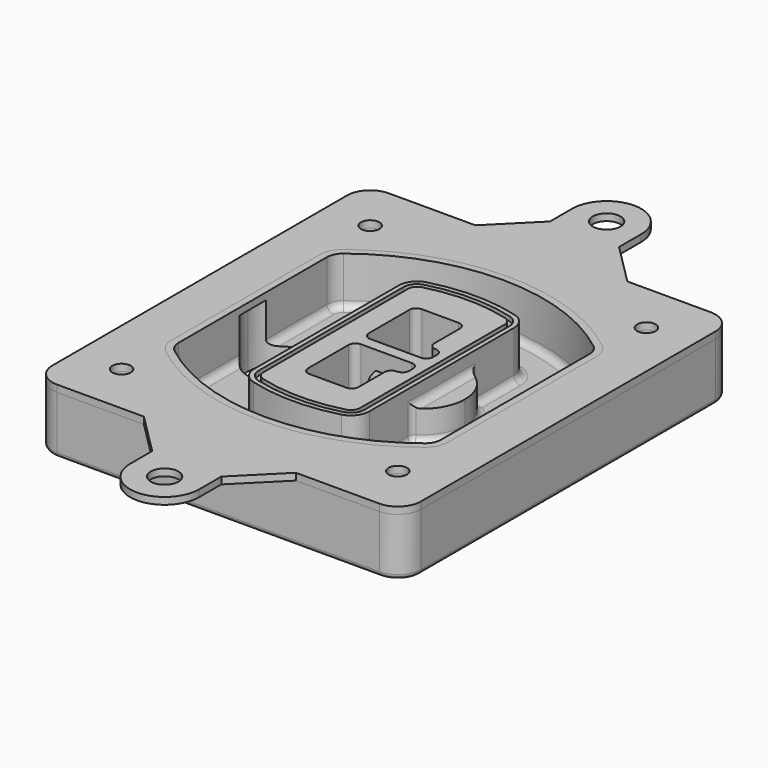
from build123d import *

# Parameters (mm, degrees)
F0_R      = 4
F1_DEPTH  = 25
F2_DEPTH  = 3
F3_DEPTH  = 18
F5_DEPTH  = 21
F6_DEPTH  = 2
F8_DEPTH  = 20
F9_DEPTH  = 16
F10_DEPTH = 25
F7_R      = 6
F7_R_2    = 4
F11_DEPTH = 6
F13_DEPTH = 9
F14_R     = 3
F15_R     = 2
F16_R     = 6
F16_R_2   = 4
F17_DEPTH = 3


with BuildPart() as f1:
    # F0 (on Top) → F1 (new body)
    with BuildSketch(Plane.XY):
        with BuildLine():
            ThreePointArc((14.05, 38.3825811321), (16.9789321881, 31.3115133202), (24.05, 28.3825811321))
            Line((24.05, 28.3825811321), (164.05, 28.3825811321))
            ThreePointArc((164.05, 28.3825811321), (171.1210678119, 31.3115133202), (174.05, 38.3825811321))
            Line((174.05, 38.3825811321), (174.05, 198.3825811321))
            ThreePointArc((174.05, 198.3825811321), (171.1210678119, 205.4536489439), (164.05, 208.3825811321))
            Line((164.05, 208.3825811321), (24.05, 208.3825811321))
            ThreePointArc((24.05, 208.3825811321), (16.9789321881, 205.4536489439), (14.05, 198.3825811321))
            Line((14.05, 198.3825811321), (14.05, 38.3825811321))
        make_face()
        with Locations((34.05, 50.8825811321)):
            Circle(F0_R, mode=Mode.SUBTRACT)
        with Locations((154.05, 50.8825811321)):
            Circle(F0_R, mode=Mode.SUBTRACT)
        with BuildLine():
            ThreePointArc((30.05, 158.6760234193), (31.4679615202, 164.8154295545), (35.4346153846, 169.7112011673))
            ThreePointArc((35.4346153846, 169.7112011673), (94.05, 189.8825811321), (152.6653846154, 169.7112011673))
            ThreePointArc((152.6653846154, 169.7112011673), (156.6320384798, 164.8154295545), (158.05, 158.6760234193))
            Line((158.05, 158.6760234193), (158.05, 78.0891388448))
            ThreePointArc((158.05, 78.0891388448), (156.6320384798, 71.9497327097), (152.6653846154, 67.0539610969))
            ThreePointArc((152.6653846154, 67.0539610969), (94.05, 46.8825811321), (35.4346153846, 67.0539610969))
            ThreePointArc((35.4346153846, 67.0539610969), (31.4679615202, 71.9497327097), (30.05, 78.0891388448))
            Line((30.05, 78.0891388448), (30.05, 158.6760234193))
        make_face(mode=Mode.SUBTRACT)
        with Locations((34.05, 185.8825811321)):
            Circle(F0_R, mode=Mode.SUBTRACT)
        with Locations((154.05, 185.8825811321)):
            Circle(F0_R, mode=Mode.SUBTRACT)
        with BuildLine():
            ThreePointArc((152.6653846154, 169.7112011673), (94.05, 189.8825811321), (35.4346153846, 169.7112011673))
            ThreePointArc((35.4346153846, 169.7112011673), (31.4679615202, 164.8154295545), (30.05, 158.6760234193))
            Line((30.05, 158.6760234193), (30.05, 78.0891388448))
            ThreePointArc((30.05, 78.0891388448), (31.4679615202, 71.9497327097), (35.4346153846, 67.0539610969))
            ThreePointArc((35.4346153846, 67.0539610969), (94.05, 46.8825811321), (152.6653846154, 67.0539610969))
            ThreePointArc((152.6653846154, 67.0539610969), (156.6320384798, 71.9497327097), (158.05, 78.0891388448))
            Line((158.05, 78.0891388448), (158.05, 158.6760234193))
            ThreePointArc((158.05, 158.6760234193), (156.6320384798, 164.8154295545), (152.6653846154, 169.7112011673))
        make_face()
        with BuildLine():
            Line((34.05, 78.0891388448), (34.05, 158.6760234193))
            ThreePointArc((34.05, 158.6760234193), (35.0628296573, 163.0613135158), (37.8961538462, 166.5582932393))
            ThreePointArc((37.8961538462, 166.5582932393), (94.05, 185.8825811321), (150.2038461538, 166.5582932393))
            ThreePointArc((150.2038461538, 166.5582932393), (153.0371703427, 163.0613135158), (154.05, 158.6760234193))
            Line((154.05, 158.6760234193), (154.05, 78.0891388448))
            ThreePointArc((154.05, 78.0891388448), (153.0371703427, 73.7038487483), (150.2038461538, 70.2068690248))
            ThreePointArc((150.2038461538, 70.2068690248), (94.05, 50.8825811321), (37.8961538462, 70.2068690248))
            ThreePointArc((37.8961538462, 70.2068690248), (35.0628296573, 73.7038487483), (34.05, 78.0891388448))
        make_face(mode=Mode.SUBTRACT)
        with BuildLine():
            ThreePointArc((37.8961538462, 166.5582932393), (35.0628296573, 163.0613135158), (34.05, 158.6760234193))
            Line((34.05, 158.6760234193), (34.05, 78.0891388448))
            ThreePointArc((34.05, 78.0891388448), (35.0628296573, 73.7038487483), (37.8961538462, 70.2068690248))
            ThreePointArc((37.8961538462, 70.2068690248), (94.05, 50.8825811321), (150.2038461538, 70.2068690248))
            ThreePointArc((150.2038461538, 70.2068690248), (153.0371703427, 73.7038487483), (154.05, 78.0891388448))
            Line((154.05, 78.0891388448), (154.05, 158.6760234193))
            ThreePointArc((154.05, 158.6760234193), (153.0371703427, 163.0613135158), (150.2038461538, 166.5582932393))
            ThreePointArc((150.2038461538, 166.5582932393), (94.05, 185.8825811321), (37.8961538462, 166.5582932393))
        make_face()
        with BuildLine():
            ThreePointArc((148.3576923077, 164.1936122933), (150.3410192399, 161.7457264869), (151.05, 158.6760234193))
            Line((151.05, 158.6760234193), (151.05, 78.0891388448))
            ThreePointArc((151.05, 78.0891388448), (150.3410192399, 75.0194357772), (148.3576923077, 72.5715499708))
            ThreePointArc((148.3576923077, 72.5715499708), (94.05, 53.8825811321), (39.7423076923, 72.5715499708))
            ThreePointArc((39.7423076923, 72.5715499708), (37.7589807601, 75.0194357772), (37.05, 78.0891388448))
            Line((37.05, 78.0891388448), (37.05, 158.6760234193))
            ThreePointArc((37.05, 158.6760234193), (37.7589807601, 161.7457264869), (39.7423076923, 164.1936122933))
            ThreePointArc((39.7423076923, 164.1936122933), (94.05, 182.8825811321), (148.3576923077, 164.1936122933))
        make_face(mode=Mode.SUBTRACT)
        with BuildLine():
            Line((151.05, 78.0891388448), (151.05, 158.6760234193))
            ThreePointArc((151.05, 158.6760234193), (150.3410192399, 161.7457264869), (148.3576923077, 164.1936122933))
            ThreePointArc((148.3576923077, 164.1936122933), (94.05, 182.8825811321), (39.7423076923, 164.1936122933))
            ThreePointArc((39.7423076923, 164.1936122933), (37.7589807601, 161.7457264869), (37.05, 158.6760234193))
            Line((37.05, 158.6760234193), (37.05, 78.0891388448))
            ThreePointArc((37.05, 78.0891388448), (37.7589807601, 75.0194357772), (39.7423076923, 72.5715499708))
            ThreePointArc((39.7423076923, 72.5715499708), (94.05, 53.8825811321), (148.3576923077, 72.5715499708))
            ThreePointArc((148.3576923077, 72.5715499708), (150.3410192399, 75.0194357772), (151.05, 78.0891388448))
        make_face()
    extrude(amount=-F1_DEPTH)

    # F0 (on Top) → F2 (join)
    with BuildSketch(Plane.XY):
        with BuildLine():
            ThreePointArc((37.8961538462, 166.5582932393), (35.0628296573, 163.0613135158), (34.05, 158.6760234193))
            Line((34.05, 158.6760234193), (34.05, 78.0891388448))
            ThreePointArc((34.05, 78.0891388448), (35.0628296573, 73.7038487483), (37.8961538462, 70.2068690248))
            ThreePointArc((37.8961538462, 70.2068690248), (94.05, 50.8825811321), (150.2038461538, 70.2068690248))
            ThreePointArc((150.2038461538, 70.2068690248), (153.0371703427, 73.7038487483), (154.05, 78.0891388448))
            Line((154.05, 78.0891388448), (154.05, 158.6760234193))
            ThreePointArc((154.05, 158.6760234193), (153.0371703427, 163.0613135158), (150.2038461538, 166.5582932393))
            ThreePointArc((150.2038461538, 166.5582932393), (94.05, 185.8825811321), (37.8961538462, 166.5582932393))
        make_face()
        with BuildLine():
            ThreePointArc((148.3576923077, 164.1936122933), (150.3410192399, 161.7457264869), (151.05, 158.6760234193))
            Line((151.05, 158.6760234193), (151.05, 78.0891388448))
            ThreePointArc((151.05, 78.0891388448), (150.3410192399, 75.0194357772), (148.3576923077, 72.5715499708))
            ThreePointArc((148.3576923077, 72.5715499708), (94.05, 53.8825811321), (39.7423076923, 72.5715499708))
            ThreePointArc((39.7423076923, 72.5715499708), (37.7589807601, 75.0194357772), (37.05, 78.0891388448))
            Line((37.05, 78.0891388448), (37.05, 158.6760234193))
            ThreePointArc((37.05, 158.6760234193), (37.7589807601, 161.7457264869), (39.7423076923, 164.1936122933))
            ThreePointArc((39.7423076923, 164.1936122933), (94.05, 182.8825811321), (148.3576923077, 164.1936122933))
        make_face(mode=Mode.SUBTRACT)
    extrude(amount=F2_DEPTH)

    # F0 (on Top) → F3 (cut)
    with BuildSketch(Plane.XY):
        with BuildLine():
            Line((151.05, 78.0891388448), (151.05, 158.6760234193))
            ThreePointArc((151.05, 158.6760234193), (150.3410192399, 161.7457264869), (148.3576923077, 164.1936122933))
            ThreePointArc((148.3576923077, 164.1936122933), (94.05, 182.8825811321), (39.7423076923, 164.1936122933))
            ThreePointArc((39.7423076923, 164.1936122933), (37.7589807601, 161.7457264869), (37.05, 158.6760234193))
            Line((37.05, 158.6760234193), (37.05, 78.0891388448))
            ThreePointArc((37.05, 78.0891388448), (37.7589807601, 75.0194357772), (39.7423076923, 72.5715499708))
            ThreePointArc((39.7423076923, 72.5715499708), (94.05, 53.8825811321), (148.3576923077, 72.5715499708))
            ThreePointArc((148.3576923077, 72.5715499708), (150.3410192399, 75.0194357772), (151.05, 78.0891388448))
        make_face()
    extrude(amount=-F3_DEPTH, mode=Mode.SUBTRACT)

    # F4 (on face) → F5 (join, through all)
    with BuildSketch(Plane.XY.offset(3)):
        with BuildLine():
            ThreePointArc((69.05, 79.13605345), (70.6988454002, 74.2716074127), (74.9657088123, 71.4123412437))
            ThreePointArc((74.9657088123, 71.4123412437), (94.05, 68.8825811321), (113.1342911877, 71.4123412437))
            ThreePointArc((113.1342911877, 71.4123412437), (117.4011545998, 74.2716074127), (119.05, 79.13605345))
            Line((119.05, 79.13605345), (119.05, 157.6291088141))
            ThreePointArc((119.05, 157.6291088141), (117.4011545998, 162.4935548514), (113.1342911877, 165.3528210204))
            ThreePointArc((113.1342911877, 165.3528210204), (94.05, 167.8825811321), (74.9657088123, 165.3528210204))
            ThreePointArc((74.9657088123, 165.3528210204), (70.6988454002, 162.4935548514), (69.05, 157.6291088141))
            Line((69.05, 157.6291088141), (69.05, 79.13605345))
        make_face()
        with BuildLine():
            ThreePointArc((112.6132183908, 163.4218929688), (115.8133659499, 161.2774433421), (117.05, 157.6291088141))
            Line((117.05, 157.6291088141), (117.05, 79.13605345))
            ThreePointArc((117.05, 79.13605345), (115.8133659499, 75.4877189221), (112.6132183908, 73.3432692953))
            ThreePointArc((112.6132183908, 73.3432692953), (94.05, 70.8825811321), (75.4867816092, 73.3432692953))
            ThreePointArc((75.4867816092, 73.3432692953), (72.2866340501, 75.4877189221), (71.05, 79.13605345))
            Line((71.05, 79.13605345), (71.05, 157.6291088141))
            ThreePointArc((71.05, 157.6291088141), (72.2866340501, 161.2774433421), (75.4867816092, 163.4218929688))
            ThreePointArc((75.4867816092, 163.4218929688), (94.05, 165.8825811321), (112.6132183908, 163.4218929688))
        make_face(mode=Mode.SUBTRACT)
        with BuildLine():
            Line((117.05, 79.13605345), (117.05, 157.6291088141))
            ThreePointArc((117.05, 157.6291088141), (115.8133659499, 161.2774433421), (112.6132183908, 163.4218929688))
            ThreePointArc((112.6132183908, 163.4218929688), (94.05, 165.8825811321), (75.4867816092, 163.4218929688))
            ThreePointArc((75.4867816092, 163.4218929688), (72.2866340501, 161.2774433421), (71.05, 157.6291088141))
            Line((71.05, 157.6291088141), (71.05, 79.13605345))
            ThreePointArc((71.05, 79.13605345), (72.2866340501, 75.4877189221), (75.4867816092, 73.3432692953))
            ThreePointArc((75.4867816092, 73.3432692953), (94.05, 70.8825811321), (112.6132183908, 73.3432692953))
            ThreePointArc((112.6132183908, 73.3432692953), (115.8133659499, 75.4877189221), (117.05, 79.13605345))
        make_face()
        with BuildLine():
            ThreePointArc((112.0921455939, 161.4909649173), (114.2255772999, 160.0613318328), (115.05, 157.6291088141))
            Line((115.05, 157.6291088141), (115.05, 79.13605345))
            ThreePointArc((115.05, 79.13605345), (114.2255772999, 76.7038304314), (112.0921455939, 75.2741973469))
            ThreePointArc((112.0921455939, 75.2741973469), (94.05, 72.8825811321), (76.0078544061, 75.2741973469))
            ThreePointArc((76.0078544061, 75.2741973469), (73.8744227001, 76.7038304314), (73.05, 79.13605345))
            Line((73.05, 79.13605345), (73.05, 157.6291088141))
            ThreePointArc((73.05, 157.6291088141), (73.8744227001, 160.0613318328), (76.0078544061, 161.4909649173))
            ThreePointArc((76.0078544061, 161.4909649173), (94.05, 163.8825811321), (112.0921455939, 161.4909649173))
        make_face(mode=Mode.SUBTRACT)
        with BuildLine():
            Line((115.05, 79.13605345), (115.05, 157.6291088141))
            ThreePointArc((115.05, 157.6291088141), (114.2255772999, 160.0613318328), (112.0921455939, 161.4909649173))
            ThreePointArc((112.0921455939, 161.4909649173), (94.05, 163.8825811321), (76.0078544061, 161.4909649173))
            ThreePointArc((76.0078544061, 161.4909649173), (73.8744227001, 160.0613318328), (73.05, 157.6291088141))
            Line((73.05, 157.6291088141), (73.05, 79.13605345))
            ThreePointArc((73.05, 79.13605345), (73.8744227001, 76.7038304314), (76.0078544061, 75.2741973469))
            ThreePointArc((76.0078544061, 75.2741973469), (94.05, 72.8825811321), (112.0921455939, 75.2741973469))
            ThreePointArc((112.0921455939, 75.2741973469), (114.2255772999, 76.7038304314), (115.05, 79.13605345))
        make_face()
        with BuildLine():
            Line((86.05, 115.8825811321), (108.05, 115.8825811321))
            ThreePointArc((108.05, 115.8825811321), (110.1713203436, 115.0039014756), (111.05, 112.8825811321))
            Line((111.05, 112.8825811321), (111.05, 110.8825811321))
            ThreePointArc((111.05, 110.8825811321), (110.1713203436, 108.7612607885), (108.05, 107.8825811321))
            ThreePointArc((108.05, 107.8825811321), (105.9286796564, 107.0039014756), (105.05, 104.8825811321))
            Line((105.05, 104.8825811321), (105.05, 90.8825811321))
            ThreePointArc((105.05, 90.8825811321), (104.1713203436, 88.7612607885), (102.05, 87.8825811321))
            Line((102.05, 87.8825811321), (86.05, 87.8825811321))
            ThreePointArc((86.05, 87.8825811321), (83.9286796564, 88.7612607885), (83.05, 90.8825811321))
            Line((83.05, 90.8825811321), (83.05, 112.8825811321))
            ThreePointArc((83.05, 112.8825811321), (83.9286796564, 115.0039014756), (86.05, 115.8825811321))
        make_face(mode=Mode.SUBTRACT)
        with BuildLine():
            ThreePointArc((86.05, 120.8825811321), (83.9286796564, 121.7612607885), (83.05, 123.8825811321))
            Line((83.05, 123.8825811321), (83.05, 145.8825811321))
            ThreePointArc((83.05, 145.8825811321), (83.9286796564, 148.0039014756), (86.05, 148.8825811321))
            Line((86.05, 148.8825811321), (102.05, 148.8825811321))
            ThreePointArc((102.05, 148.8825811321), (104.1713203436, 148.0039014756), (105.05, 145.8825811321))
            Line((105.05, 145.8825811321), (105.05, 131.8825811321))
            ThreePointArc((105.05, 131.8825811321), (105.9286796564, 129.7612607885), (108.05, 128.8825811321))
            ThreePointArc((108.05, 128.8825811321), (110.1713203436, 128.0039014756), (111.05, 125.8825811321))
            Line((111.05, 125.8825811321), (111.05, 123.8825811321))
            ThreePointArc((111.05, 123.8825811321), (110.1713203436, 121.7612607885), (108.05, 120.8825811321))
            Line((108.05, 120.8825811321), (86.05, 120.8825811321))
        make_face(mode=Mode.SUBTRACT)
    extrude(amount=-F5_DEPTH)

    # F4 (on face) → F6 (cut)
    with BuildSketch(Plane.XY.offset(3)):
        with BuildLine():
            Line((117.05, 79.13605345), (117.05, 157.6291088141))
            ThreePointArc((117.05, 157.6291088141), (115.8133659499, 161.2774433421), (112.6132183908, 163.4218929688))
            ThreePointArc((112.6132183908, 163.4218929688), (94.05, 165.8825811321), (75.4867816092, 163.4218929688))
            ThreePointArc((75.4867816092, 163.4218929688), (72.2866340501, 161.2774433421), (71.05, 157.6291088141))
            Line((71.05, 157.6291088141), (71.05, 79.13605345))
            ThreePointArc((71.05, 79.13605345), (72.2866340501, 75.4877189221), (75.4867816092, 73.3432692953))
            ThreePointArc((75.4867816092, 73.3432692953), (94.05, 70.8825811321), (112.6132183908, 73.3432692953))
            ThreePointArc((112.6132183908, 73.3432692953), (115.8133659499, 75.4877189221), (117.05, 79.13605345))
        make_face()
        with BuildLine():
            ThreePointArc((112.0921455939, 161.4909649173), (114.2255772999, 160.0613318328), (115.05, 157.6291088141))
            Line((115.05, 157.6291088141), (115.05, 79.13605345))
            ThreePointArc((115.05, 79.13605345), (114.2255772999, 76.7038304314), (112.0921455939, 75.2741973469))
            ThreePointArc((112.0921455939, 75.2741973469), (94.05, 72.8825811321), (76.0078544061, 75.2741973469))
            ThreePointArc((76.0078544061, 75.2741973469), (73.8744227001, 76.7038304314), (73.05, 79.13605345))
            Line((73.05, 79.13605345), (73.05, 157.6291088141))
            ThreePointArc((73.05, 157.6291088141), (73.8744227001, 160.0613318328), (76.0078544061, 161.4909649173))
            ThreePointArc((76.0078544061, 161.4909649173), (94.05, 163.8825811321), (112.0921455939, 161.4909649173))
        make_face(mode=Mode.SUBTRACT)
    extrude(amount=-F6_DEPTH, mode=Mode.SUBTRACT)

    # F7 (on face) → F8 (join)
    with BuildSketch(Plane(origin=(0, 0, -25), x_dir=(1, 0, 0), z_dir=(0, 0, -1))):
        with BuildLine():
            ThreePointArc((97.33842436, -118.3825811321), (110.8067035675, -104.9143019245), (124.274982775, -118.3825811321))
            Line((124.274982775, -118.3825811321), (129.274982775, -118.3825811321))
            ThreePointArc((129.274982775, -118.3825811321), (110.8067035675, -99.9143019245), (92.33842436, -118.3825811321))
            Line((92.33842436, -118.3825811321), (97.33842436, -118.3825811321))
        make_face()
        with BuildLine():
            Line((97.33842436, -118.3825811321), (124.274982775, -118.3825811321))
            ThreePointArc((124.274982775, -118.3825811321), (110.8067035675, -104.9143019245), (97.33842436, -118.3825811321))
        make_face()
        with BuildLine():
            ThreePointArc((97.33842436, -118.3825811321), (110.8067035675, -131.8508603396), (124.274982775, -118.3825811321))
            Line((124.274982775, -118.3825811321), (97.33842436, -118.3825811321))
        make_face()
        with BuildLine():
            Line((129.274982775, -118.3825811321), (124.274982775, -118.3825811321))
            ThreePointArc((124.274982775, -118.3825811321), (110.8067035675, -131.8508603396), (97.33842436, -118.3825811321))
            Line((97.33842436, -118.3825811321), (92.33842436, -118.3825811321))
            ThreePointArc((92.33842436, -118.3825811321), (110.8067035675, -136.8508603396), (129.274982775, -118.3825811321))
        make_face()
    extrude(amount=-F8_DEPTH)

    # F7 (on face) → F9 (cut)
    with BuildSketch(Plane(origin=(0, 0, -25), x_dir=(1, 0, 0), z_dir=(0, 0, -1))):
        with BuildLine():
            Line((97.33842436, -118.3825811321), (124.274982775, -118.3825811321))
            ThreePointArc((124.274982775, -118.3825811321), (110.8067035675, -104.9143019245), (97.33842436, -118.3825811321))
        make_face()
        with BuildLine():
            ThreePointArc((97.33842436, -118.3825811321), (110.8067035675, -131.8508603396), (124.274982775, -118.3825811321))
            Line((124.274982775, -118.3825811321), (97.33842436, -118.3825811321))
        make_face()
    extrude(amount=-F9_DEPTH, mode=Mode.SUBTRACT)

    # F7 (on face) → F10 (cut)
    with BuildSketch(Plane(origin=(0, 0, -25), x_dir=(1, 0, 0), z_dir=(0, 0, -1))):
        with BuildLine():
            Line((35.0181770675, -118.3825811321), (61.9547354825, -118.3825811321))
            ThreePointArc((61.9547354825, -118.3825811321), (48.486456275, -104.9143019245), (35.0181770675, -118.3825811321))
        make_face()
        with BuildLine():
            ThreePointArc((35.0181770675, -118.3825811321), (48.486456275, -131.8508603396), (61.9547354825, -118.3825811321))
            Line((61.9547354825, -118.3825811321), (35.0181770675, -118.3825811321))
        make_face()
    extrude(amount=-F10_DEPTH, mode=Mode.SUBTRACT)

    # F7 (on face) → F11 (cut)
    with BuildSketch(Plane(origin=(0, 0, -25), x_dir=(1, 0, 0), z_dir=(0, 0, -1))):
        with Locations((154.05, -185.8825811321)):
            Circle(F7_R)
        with Locations((154.05, -185.8825811321)):
            Circle(F7_R_2, mode=Mode.SUBTRACT)
        with Locations((34.05, -185.8825811321)):
            Circle(F7_R)
        with Locations((34.05, -185.8825811321)):
            Circle(F7_R_2, mode=Mode.SUBTRACT)
        with Locations((34.05, -50.8825811321)):
            Circle(F7_R)
        with Locations((34.05, -50.8825811321)):
            Circle(F7_R_2, mode=Mode.SUBTRACT)
        with Locations((154.05, -50.8825811321)):
            Circle(F7_R)
        with Locations((154.05, -50.8825811321)):
            Circle(F7_R_2, mode=Mode.SUBTRACT)
    extrude(amount=-F11_DEPTH, mode=Mode.SUBTRACT)

    # F12 (on face) → F13 (cut, through all)
    with BuildSketch(Plane(origin=(0, 0, -9), x_dir=(1, 0, 0), z_dir=(0, 0, -1))):
        with BuildLine():
            Line((105.05, -104.8825811321), (105.05, -100.8344273567))
            ThreePointArc((105.05, -100.8344273567), (96.6196536419, -106.5586667507), (92.5084157545, -115.8825811321))
            Line((92.5084157545, -115.8825811321), (97.5724848595, -115.8825811321))
            ThreePointArc((97.5724848595, -115.8825811321), (100.2357188154, -110.0369939039), (105.3036447004, -106.0898642673))
            ThreePointArc((105.3036447004, -106.0898642673), (105.1140958889, -105.4994012441), (105.05, -104.8825811321))
        make_face()
        with BuildLine():
            ThreePointArc((105.3036447004, -130.6752979968), (100.2357188154, -126.7281683602), (97.5724848595, -120.8825811321))
            Line((97.5724848595, -120.8825811321), (92.5084157545, -120.8825811321))
            ThreePointArc((92.5084157545, -120.8825811321), (96.6196536419, -130.2064955134), (105.05, -135.9307349074))
            Line((105.05, -135.9307349074), (105.05, -131.8825811321))
            ThreePointArc((105.05, -131.8825811321), (105.1140958889, -131.26576102), (105.3036447004, -130.6752979968))
        make_face()
        with BuildLine():
            ThreePointArc((105.3036447004, -106.0898642673), (100.2357188154, -110.0369939039), (97.5724848595, -115.8825811321))
            Line((97.5724848595, -115.8825811321), (108.05, -115.8825811321))
            ThreePointArc((108.05, -115.8825811321), (110.1713203436, -115.0039014756), (111.05, -112.8825811321))
            Line((111.05, -112.8825811321), (111.05, -110.8825811321))
            ThreePointArc((111.05, -110.8825811321), (110.1713203436, -108.7612607885), (108.05, -107.8825811321))
            ThreePointArc((108.05, -107.8825811321), (106.4101599782, -107.3947365219), (105.3036447004, -106.0898642673))
        make_face()
        with BuildLine():
            Line((108.05, -120.8825811321), (97.5724848595, -120.8825811321))
            ThreePointArc((97.5724848595, -120.8825811321), (100.2357188154, -126.7281683602), (105.3036447004, -130.6752979968))
            ThreePointArc((105.3036447004, -130.6752979968), (106.4101599782, -129.3704257422), (108.05, -128.8825811321))
            ThreePointArc((108.05, -128.8825811321), (110.1713203436, -128.0039014756), (111.05, -125.8825811321))
            Line((111.05, -125.8825811321), (111.05, -123.8825811321))
            ThreePointArc((111.05, -123.8825811321), (110.1713203436, -121.7612607885), (108.05, -120.8825811321))
        make_face()
    extrude(amount=F13_DEPTH, mode=Mode.SUBTRACT)

    # F14
    f14_edges = [f1.edges().sort_by_distance(p)[0] for p in [
        (37.05, 94.679105, -18),
        (37.05, 142.086057, -18),
        (119.05, 118.382581, -5),
        (119.05, 134.909087, -11.5),
        (119.05, 101.856075, -11.5),
        (119.05, 90.496064, -18),
        (129.274983, 118.382581, -18),
    ]]
    fillet(f14_edges, radius=F14_R)

    # F15
    f15_edges = [f1.edges().sort_by_distance(p)[0] for p in [
        (94.05, 28.382581, -25),
    ]]
    fillet(f15_edges, radius=F15_R)


with BuildPart() as f17:
    # F16 (on face) → F17 (new body, through all)
    with BuildSketch(Plane.XY):
        with BuildLine():
            Line((79.7550348938, 226.3825811321), (61.7550348938, 208.3825811321))
            Line((61.7550348938, 208.3825811321), (127.7550348938, 208.3825811321))
            Line((127.7550348938, 208.3825811321), (109.7550348938, 226.3825811321))
            Line((109.7550348938, 226.3825811321), (109.7550348938, 238.3825811321))
            ThreePointArc((109.7550348938, 238.3825811321), (94.7550348938, 253.3825811321), (79.7550348938, 238.3825811321))
            Line((79.7550348938, 238.3825811321), (79.7550348938, 226.3825811321))
        make_face()
        with Locations((94.7550348938, 238.3825811321)):
            Circle(F16_R, mode=Mode.SUBTRACT)
        with BuildLine():
            Line((127.7550348938, 28.3825811321), (61.7550348938, 28.3825811321))
            Line((61.7550348938, 28.3825811321), (79.7550348938, 10.3825811321))
            Line((79.7550348938, 10.3825811321), (79.7550348938, -1.6174188679))
            ThreePointArc((79.7550348938, -1.6174188679), (94.7550348938, -16.6174188679), (109.7550348938, -1.6174188679))
            Line((109.7550348938, -1.6174188679), (109.7550348938, 10.3825811321))
            Line((109.7550348938, 10.3825811321), (127.7550348938, 28.3825811321))
        make_face()
        with Locations((94.7550348938, -1.6174188679)):
            Circle(F16_R, mode=Mode.SUBTRACT)
        with BuildLine():
            Line((127.7550348938, 208.3825811321), (61.7550348938, 208.3825811321))
            Line((61.7550348938, 208.3825811321), (24.05, 208.3825811321))
            ThreePointArc((24.05, 208.3825811321), (16.9789321881, 205.4536489439), (14.05, 198.3825811321))
            Line((14.05, 198.3825811321), (14.05, 38.3825811321))
            ThreePointArc((14.05, 38.3825811321), (16.9789321881, 31.3115133202), (24.05, 28.3825811321))
            Line((24.05, 28.3825811321), (61.7550348938, 28.3825811321))
            Line((61.7550348938, 28.3825811321), (127.7550348938, 28.3825811321))
            Line((127.7550348938, 28.3825811321), (164.05, 28.3825811321))
            ThreePointArc((164.05, 28.3825811321), (171.1210678119, 31.3115133202), (174.05, 38.3825811321))
            Line((174.05, 38.3825811321), (174.05, 198.3825811321))
            ThreePointArc((174.05, 198.3825811321), (171.1210678119, 205.4536489439), (164.05, 208.3825811321))
            Line((164.05, 208.3825811321), (127.7550348938, 208.3825811321))
        make_face()
        with Locations((34.05, 50.8825811321)):
            Circle(F16_R_2, mode=Mode.SUBTRACT)
        with Locations((154.05, 50.8825811321)):
            Circle(F16_R_2, mode=Mode.SUBTRACT)
        with Locations((34.05, 185.8825811321)):
            Circle(F16_R_2, mode=Mode.SUBTRACT)
        with BuildLine():
            ThreePointArc((34.05, 158.6760234193), (35.0628296573, 163.0613135158), (37.8961538462, 166.5582932393))
            ThreePointArc((37.8961538462, 166.5582932393), (94.05, 185.8825811321), (150.2038461538, 166.5582932393))
            ThreePointArc((150.2038461538, 166.5582932393), (153.0371703427, 163.0613135158), (154.05, 158.6760234193))
            Line((154.05, 158.6760234193), (154.05, 78.0891388448))
            ThreePointArc((154.05, 78.0891388448), (153.0371703427, 73.7038487483), (150.2038461538, 70.2068690248))
            ThreePointArc((150.2038461538, 70.2068690248), (94.05, 50.8825811321), (37.8961538462, 70.2068690248))
            ThreePointArc((37.8961538462, 70.2068690248), (35.0628296573, 73.7038487483), (34.05, 78.0891388448))
            Line((34.05, 78.0891388448), (34.05, 158.6760234193))
        make_face(mode=Mode.SUBTRACT)
        with Locations((154.05, 185.8825811321)):
            Circle(F16_R_2, mode=Mode.SUBTRACT)
    extrude(amount=F17_DEPTH)


solid = Compound([f1.part, f17.part])
